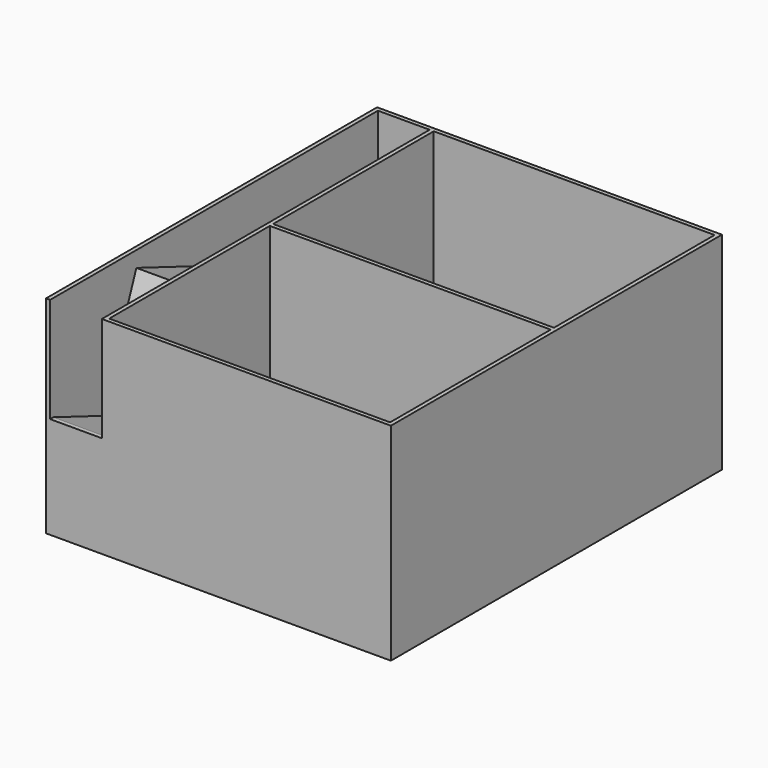
from build123d import *

# Parameters (mm, degrees)
F0_W      = 127
F0_H      = 152.4
F1_DEPTH  = 76.2
F2_T      = -1.4986
F3_W      = 1.4986
F3_H      = 149.4028
F4_DEPTH  = 74.7014
F5_W      = 103.4542
F5_H      = 1.4986
F6_DEPTH  = 74.7014
F8_DEPTH  = 20.5486
F9_W      = 19.05
F9_H      = 38.6785856472
F10_DEPTH = 4.064


# Not quite as in the source:
# - an extrude ends at something that could not be found from the text; its depth is read off the source's solid


with BuildPart() as f1:
    # F0 (on Top) → F1 (new body)
    with BuildSketch(Plane.XY):
        Rectangle(F0_W, F0_H)
    extrude(amount=F1_DEPTH)

    # F2
    f2_openings = [f1.faces().sort_by_distance(p)[0] for p in [
        (0, 0, 76.2),
    ]]
    offset(amount=F2_T, openings=f2_openings)

    # F3 (on face) → F4 (join, through all)
    with BuildSketch(Plane.XY.offset(1.4986)):
        with Locations((-42.2021, 0)):
            Rectangle(F3_W, F3_H)
    extrude(amount=F4_DEPTH)

    # F5 (on face) → F6 (join, through all)
    with BuildSketch(Plane.XY.offset(1.4986)):
        with Locations((10.2743, 0)):
            Rectangle(F5_W, F5_H)
    extrude(amount=F6_DEPTH)

    # F7 (on face) → F8 (join, through all)
    with BuildSketch(Plane(origin=(-63.5, 0, 0), x_dir=(0, -1, 0), z_dir=(-1, 0, 0))):
        Polygon((76.2, 0), (76.2, 38.1), (52.5047014133, 28.9516217345), (36.4950394487, 70.4183942612), (-76.2, 26.9086302568), (-76.2, 0), align=None)
    extrude(amount=-F8_DEPTH)

    # F9 (on face) → F10 (cut)
    with BuildSketch(Plane(origin=(0, -74.7014, 0), x_dir=(-1, 0, 0), z_dir=(0, 1, 0))):
        with Locations((52.4764, 56.8607071764)):
            Rectangle(F9_W, F9_H)
    extrude(amount=-F10_DEPTH, mode=Mode.SUBTRACT)


solid = f1.part
